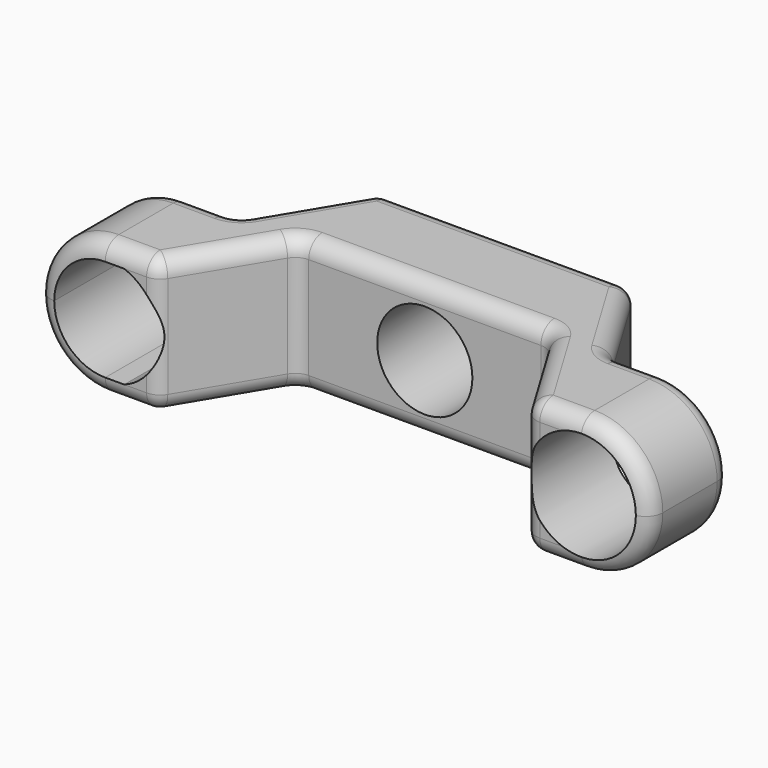
from build123d import *

# Parameters (mm, degrees)
F1_DEPTH = 40
F2_R     = 19.99999
F3_F1_R  = 5
F3_F2_R  = 5
F4_R     = 16
F4_R_2   = 14
F5_DEPTH = 66.5


# Not quite as in the source:
# - a fillet or chamfer is up to 0.001 mm smaller than in the source, because OpenCascade refuses the exact size
# - ends of sketch curves that miss each other by under 0.0002 mm in the source are joined


with BuildPart() as f1:
    # F0 (on Top) → F1 (new body)
    with BuildSketch(Plane.XY):
        Polygon((-72.9024875954, 30), (-72.9024875954, 0), (-37.9024875954, 0), (-19.8747312181, 30), (17.0975124046, 30), (54.0697560273, 30), (72.0975124046, 0), (107.0975124046, 0), (107.0975124046, 30), (72.0975124046, 30), (54.0697560273, 60), (17.0975124046, 60), (-19.8747312181, 60), (-37.9024875954, 30), align=None)
    extrude(amount=F1_DEPTH)

    # F2 (radius 20 in the source; OpenCascade refuses exactly that, so slightly less here)
    f2_edges = [f1.edges().sort_by_distance(p)[0] for p in [
        (-72.902488, 15, 40),
        (-72.902488, 15, 0),
        (107.097512, 15, 40),
        (107.097512, 15, 0),
    ]]
    fillet(f2_edges, radius=F2_R)

    # F3: fillet of radius 5 on 16 edges, made by hand

    # F3_f1
    f3_f1_edges = [f1.edges().sort_by_distance(p)[0] for p in [
        (-19.8747312181, 30, 20),
        (54.0697560273, 30, 20),
        (72.0975124046, 30, 20),
        (-37.9024875954, 30, 20),
    ]]
    fillet(f3_f1_edges, radius=F3_F1_R)

    # F3_f2
    f3_f2_edges = [f1.edges().sort_by_distance(p)[0] for p in [
        (-37.9024875954, 0, 20),
        (72.0975124046, 0, 20),
        (54.0697560273, 60, 20),
        (-19.8747312181, 60, 20),
        (62.3551307083, 46.2123031159, 40),
        (17.0975124046, 60, 40),
        (-28.1601058991, 46.2123031159, 40),
        (63.8121377235, 13.7876968841, 40),
        (101.2396509572, 0, 5.8578614473),
        (-67.0446261481, 0, 5.8578614473),
        (17.0975124046, 30, 0),
        (17.0975124046, 60, 0),
        (-72.9024875954, 0, 20),
        (-45.4024925954, 0, 0),
        (-67.0446261481, 0, 34.1421385527),
        (-45.4024925954, 0, 40),
        (107.0975124046, 0, 20),
        (79.5975174046, 0, 0),
        (101.2396509572, 0, 34.1421385527),
        (79.5975174046, 0, 40),
        (-19.5080384845, 29.3518369019, 0),
        (53.7030632936, 29.3518369019, 0),
        (53.7030632936, 29.3518369019, 40),
        (-38.269180329, 30.6481630981, 40),
        (72.4642051382, 30.6481630981, 40),
    ]]
    fillet(f3_f2_edges, radius=F3_F2_R)

    # F4 (on face) → F5 (cut)
    with BuildSketch(Plane.XZ):
        with BuildLine():
            Line((-40.7311948659, 9.6144507468), (-40.7311948659, 30.3855492532))
            ThreePointArc((-40.7311948659, 30.3855492532), (-43.7377821689, 33.1151886927), (-47.3347232326, 35))
            Line((-47.3347232326, 35), (-52.9024975954, 35))
            ThreePointArc((-52.9024975954, 35), (-63.5090922422, 30.6066046467), (-67.9024875954, 20.00001))
            ThreePointArc((-67.9024875954, 20.00001), (-63.5090922422, 9.3933953533), (-52.9024975954, 5))
            Line((-52.9024975954, 5), (-47.3347232326, 5))
            ThreePointArc((-47.3347232326, 5), (-43.7377821689, 6.8848113073), (-40.7311948659, 9.6144507468))
        make_face()
        with Locations((87.0975124046, 20)):
            Circle(F4_R)
        with BuildLine():
            ThreePointArc((-40.7311948659, 9.6144507468), (-37.8901479431, 14.4655932419), (-36.9024875954, 20))
            ThreePointArc((-36.9024875954, 20), (-37.8901479431, 25.5344067581), (-40.7311948659, 30.3855492532))
            Line((-40.7311948659, 30.3855492532), (-40.7311948659, 9.6144507468))
        make_face()
        with Locations((17.0975124046, 20)):
            Circle(F4_R_2)
    extrude(amount=-F5_DEPTH, mode=Mode.SUBTRACT)


solid = f1.part
